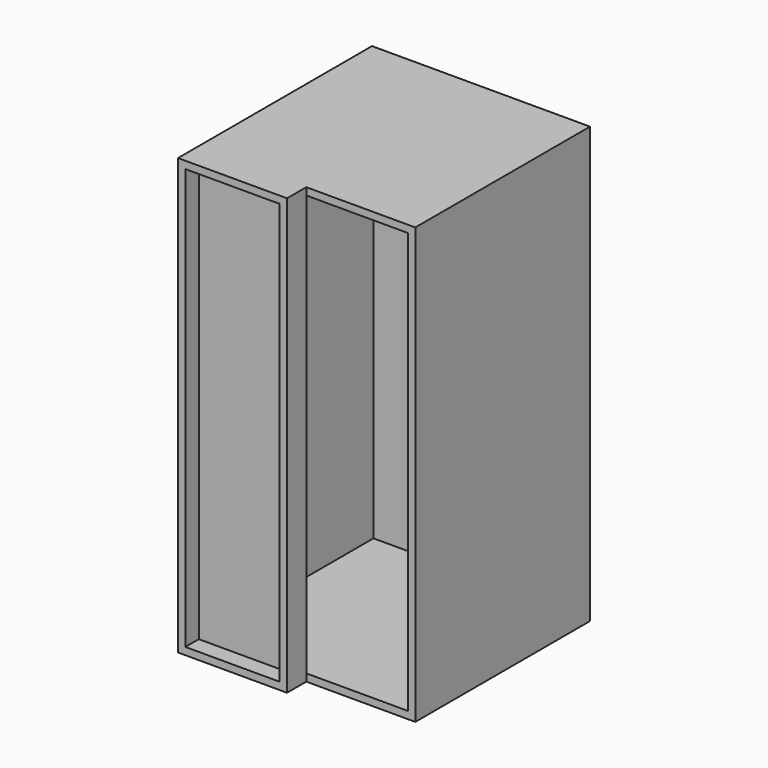
from build123d import *

# Parameters (mm, degrees)
F0_W         = 75.8234336972
F0_H         = 151.4142677188
F1_DEPTH     = 75.946
F3_T         = -2.54
F2_W         = 37.9117168486
F2_H         = 151.4142677188
F4_DEPTH     = 8.382
F5_T         = 2.54
F5_T3_DEPTH  = 7.62
F5_T5_DEPTH  = 7.62
F5_T7_DEPTH  = 40.4517168486
F5_T9_DEPTH  = 151.4142677188
F5_T11_DEPTH = 78.486
F5_T13_DEPTH = 75.8234336972


# Not quite as in the source:
# - a shell that OpenCascade refuses in one call is made with other operations: the cavity is built on its own and cut out


with BuildPart() as f1:
    # F0 (on Front) → F1 (new body)
    with BuildSketch(Plane.XZ):
        with Locations((-37.9117168486, -0.1162923872)):
            Rectangle(F0_W, F0_H)
    extrude(amount=F1_DEPTH)

    # F3
    f3_openings = [f1.faces().sort_by_distance(p)[0] for p in [
        (-37.911717, -75.946, -0.116292),
    ]]
    offset(amount=F3_T, openings=f3_openings)

    # F2 (on face) → F4 (join)
    with BuildSketch(Plane.XZ.offset(75.946)):
        with Locations((-56.8675752729, -0.1162923872)):
            Rectangle(F2_W, F2_H)
    extrude(amount=F4_DEPTH)

    # F5: shell of thickness 2.54, made by hand


with BuildPart() as f5_core1:
    # F5_t2: copy of F1
    add(f1.part)

    # the walls: a layer under each face that stays
    f5_faces = [f5_core1.faces().sort_by_distance(p)[0] for p in [
        (-37.9117168486, -42.164, 75.5908414721),
        (-37.9117168486, 0, -0.1162923872),
        (-37.9117168486, -42.164, -75.8234262466),
        (-75.8234336972, -42.164, -0.1162923872),
        (-37.9117168486, -80.137, -0.1162923872),
        (-55.5975752729, -75.946, -0.1162923872),
        (-37.9117168486, -39.243, 73.0508414721),
        (-2.54, -39.243, -0.1162923872),
        (-37.9117168486, -2.54, -0.1162923872),
        (-73.2834336972, -39.243, -0.1162923872),
        (-37.9117168486, -39.243, -73.2834262466),
        (-1.263723895, -75.946, -70.7762839894),
        (0, -37.973, -0.1162923872),
    ]]
    thicken(f5_faces, amount=-F5_T, mode=Mode.SUBTRACT)

    # F5_s4 → F5_t3 (cut)
    with BuildSketch(Plane.XY.offset(-78.3634262466)):
        Polygon((-37.8863168486, -75.9714), (-40.4517168486, -75.946), (-40.4517168486, -73.406), (-37.9117168486, -73.406), align=None)
    extrude(amount=F5_T3_DEPTH, mode=Mode.SUBTRACT)

    # F5_s6 → F5_t5 (cut)
    with BuildSketch(Plane.XY.offset(70.5108414721)):
        Polygon((-37.8863168486, -75.9714), (-40.4517168486, -75.946), (-40.4517168486, -73.406), (-37.9117168486, -73.406), align=None)
    extrude(amount=F5_T5_DEPTH, mode=Mode.SUBTRACT)

    # F5_s8 → F5_t7 (cut)
    with BuildSketch(Plane.YZ.offset(-75.8234336972)):
        Polygon((-75.9206, -73.2580262466), (-78.486, -73.2834262466), (-78.486, -75.8234262466), (-75.946, -75.8234262466), align=None)
        Polygon((-75.9206, 73.0254414721), (-78.486, 73.0508414721), (-78.486, 75.5908414721), (-75.946, 75.5908414721), align=None)
    extrude(amount=F5_T7_DEPTH, mode=Mode.SUBTRACT)

    # F5_s10 → F5_t9 (cut)
    with BuildSketch(Plane.XY.offset(-75.8234262466)):
        Polygon((-73.2580336972, -75.9206), (-73.2834336972, -78.486), (-75.8234336972, -78.486), (-75.8234336972, -75.946), align=None)
        Polygon((-2.5654, -2.5654), (0, -2.54), (0, 0), (-2.54, 0), align=None)
        Polygon((-73.2580336972, -2.5654), (-73.2834336972, 0), (-75.8234336972, 0), (-75.8234336972, -2.54), align=None)
    extrude(amount=F5_T9_DEPTH, mode=Mode.SUBTRACT)

    # F5_s12 → F5_t11 (cut)
    with BuildSketch(Plane.XZ):
        Polygon((-73.2580336972, 73.0254414721), (-73.2834336972, 75.5908414721), (-75.8234336972, 75.5908414721), (-75.8234336972, 73.0508414721), align=None)
        Polygon((-2.5654, 73.0254414721), (-2.54, 75.5908414721), (0, 75.5908414721), (0, 73.0508414721), align=None)
        Polygon((-2.5654, -73.2580262466), (0, -73.2834262466), (0, -75.8234262466), (-2.54, -75.8234262466), align=None)
        Polygon((-73.2580336972, -73.2580262466), (-75.8234336972, -73.2834262466), (-75.8234336972, -75.8234262466), (-73.2834336972, -75.8234262466), align=None)
    extrude(amount=F5_T11_DEPTH, mode=Mode.SUBTRACT)

    # F5_s14 → F5_t13 (cut)
    with BuildSketch(Plane.YZ.offset(-75.8234336972)):
        Polygon((-2.5654, 73.0254414721), (-2.54, 75.5908414721), (0, 75.5908414721), (0, 73.0508414721), align=None)
        Polygon((-2.5654, -73.2580262466), (0, -73.2834262466), (0, -75.8234262466), (-2.54, -75.8234262466), align=None)
    extrude(amount=F5_T13_DEPTH, mode=Mode.SUBTRACT)


with BuildPart() as f1_1:
    add(f1.part)

    # what is left inside the walls is the cavity
    f5_cavity = [f5_core1.part.solids().sort_by_distance(p)[0] for p in [
        (-56.867575, -78.5114, -24.505337),
    ]]
    add(f5_cavity, mode=Mode.SUBTRACT)


solid = f1_1.part
